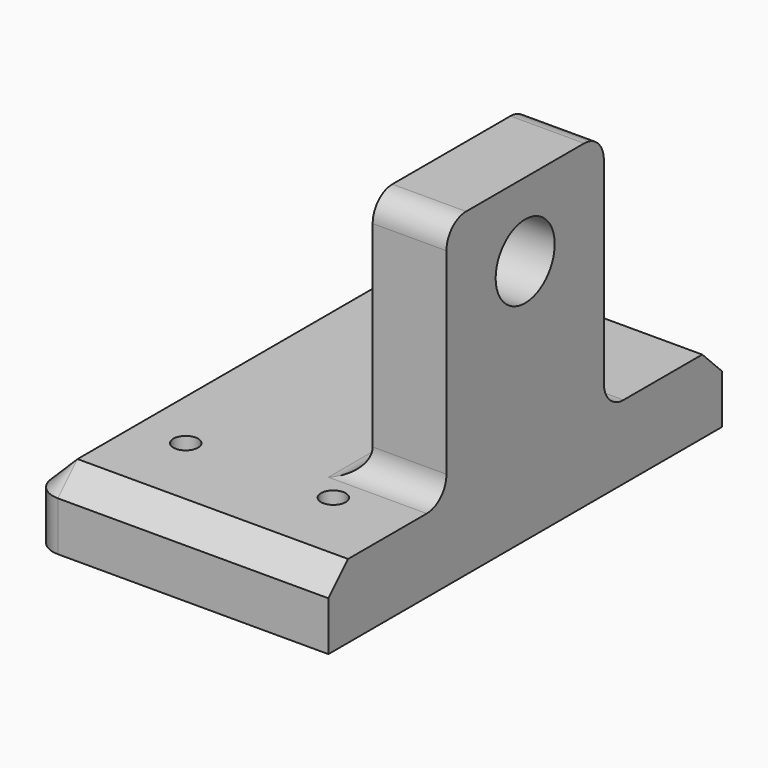
from build123d import *

# Parameters (mm, degrees)
F1_DEPTH = 15
F2_W     = 40
F2_H     = 50
F3_DEPTH = 15
F4_R     = 5
F5_SIZE  = 4.99999
F6_R     = 7.5
F7_DEPTH = 15
F8_R     = 2.5
F9_DEPTH = 15


# Not quite as in the source:
# - a fillet or chamfer is up to 0.001 mm smaller than in the source, because OpenCascade refuses the exact size


with BuildPart() as f1:
    # F0 (on Top) → F1 (new body)
    with BuildSketch(Plane.XY):
        with BuildLine():
            Line((-25, -50), (30, -50))
            Line((30, -50), (30, 50))
            Line((30, 50), (-25, 50))
            ThreePointArc((-25, 50), (-28.5355339059, 48.5355339059), (-30, 45))
            Line((-30, 45), (-30, -45))
            ThreePointArc((-30, -45), (-28.5355339059, -48.5355339059), (-25, -50))
        make_face()
    extrude(amount=F1_DEPTH)

    # F2 (on face) → F3 (join)
    with BuildSketch(Plane.YZ.offset(30)):
        with Locations((0, 40)):
            Rectangle(F2_W, F2_H)
    extrude(amount=-F3_DEPTH)

    # F4
    f4_edges = [f1.edges().sort_by_distance(p)[0] for p in [
        (22.5, -20, 15),
        (15, 0, 15),
        (22.5, 20, 15),
        (22.5, -20, 65),
        (22.5, 20, 65),
    ]]
    fillet(f4_edges, radius=F4_R)

    # F5 (size 5 in the source; OpenCascade refuses exactly that, so slightly less here)
    f5_edges = [f1.edges().sort_by_distance(p)[0] for p in [
        (2.5, 50, 15),
        (-28.535534, 48.535534, 15),
        (-30, 0, 15),
        (-28.535534, -48.535534, 15),
        (2.5, -50, 15),
    ]]
    chamfer(f5_edges, length=F5_SIZE)

    # F6 (on face) → F7 (cut, through all)
    with BuildSketch(Plane(origin=(15, 0, 0), x_dir=(0, -1, 0), z_dir=(-1, 0, 0))):
        with Locations((0, 50)):
            Circle(F6_R)
    extrude(amount=-F7_DEPTH, mode=Mode.SUBTRACT)

    # F8 (on face) → F9 (cut, through all)
    with BuildSketch(Plane(origin=(0, 0, 0), x_dir=(1, 0, 0), z_dir=(0, 0, -1))):
        with Locations((-15, -30)):
            Circle(F8_R)
        with Locations((-15, 30)):
            Circle(F8_R)
        with Locations((15, -30)):
            Circle(F8_R)
        with Locations((15, 30)):
            Circle(F8_R)
    extrude(amount=-F9_DEPTH, mode=Mode.SUBTRACT)


solid = f1.part
